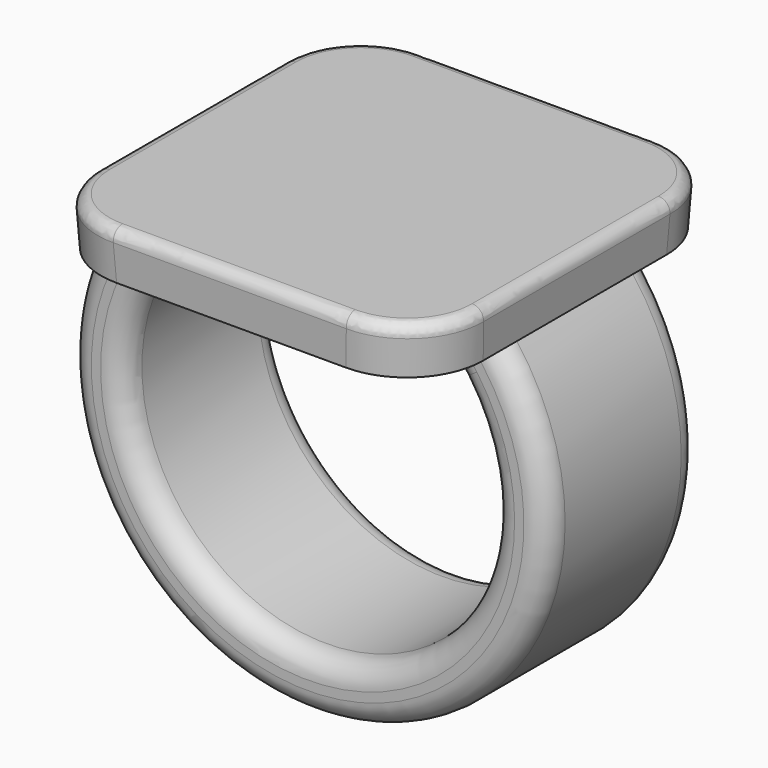
from build123d import *

# Parameters (mm, degrees)
F0_W          = 25.4
F0_H          = 25.4
F1_DEPTH      = 3.175
F1_TAPER      = -3
F3_W          = 5.08
F3_H          = 12.7
F6_DEPTH      = 6.35
F6_DEPTH_BACK = 6.35
F7_R          = 5.08
F8_R          = 1.524
F9_R          = 0.762


with BuildPart() as f1:
    # F0 (on Top) → F1 (new body)
    with BuildSketch(Plane.XY):
        Rectangle(F0_W, F0_H)
    extrude(amount=F1_DEPTH, taper=F1_TAPER)

    # F4: sweep along a path in F2
    with BuildLine(Plane.XZ) as f4_path:
        ThreePointArc((-10.16, 0), (0, -23.5582897328), (10.16, 0))
    # F3 (on face) → F4 (sweep)
    with BuildSketch(Plane(origin=(0, 0, 0), x_dir=(1, 0, 0), z_dir=(0, 0, -1))):
        with Locations((-10.16, 0)):
            Rectangle(F3_W, F3_H)
    sweep(path=f4_path.line)

    # F5 (on Front) → F6 (join, two sides)
    with BuildSketch(Plane.XZ) as f6_sk:
        with BuildLine():
            Line((10.0130578512, -2.535746045), (10.16, 0))
            Line((10.16, 0), (7.62, 0))
            ThreePointArc((7.62, 0), (8.9072265211, -1.1822790439), (10.0130578512, -2.535746045))
        make_face()
    extrude(amount=F6_DEPTH)
    extrude(f6_sk.sketch, amount=-F6_DEPTH_BACK)

    # F7
    f7_edges = [f1.edges().sort_by_distance(p)[0] for p in [
        (-12.783197, -12.783197, 1.5875),
        (-12.783197, 12.783197, 1.5875),
        (12.783197, -12.783197, 1.5875),
        (12.783197, 12.783197, 1.5875),
    ]]
    fillet(f7_edges, radius=F7_R)

    # F8
    f8_edges = [f1.edges().sort_by_distance(p)[0] for p in [
        (-1.743325, 6.35, -21.711017),
        (-1.743325, -6.35, -21.711017),
        (8.907227, -6.35, -1.182279),
        (0, 6.35, -25.501344),
        (0, -6.35, -25.501344),
        (8.907227, 6.35, -1.182279),
    ]]
    fillet(f8_edges, radius=F8_R)

    # F9
    f9_edges = [f1.edges().sort_by_distance(p)[0] for p in [
        (12.866395, 0, 3.175),
        (11.381378, -11.381378, 3.175),
        (11.381378, 11.381378, 3.175),
        (0, -12.866395, 3.175),
        (0, 12.866395, 3.175),
        (-11.381378, -11.381378, 3.175),
        (-11.381378, 11.381378, 3.175),
        (-12.866395, 0, 3.175),
    ]]
    fillet(f9_edges, radius=F9_R)


solid = f1.part
